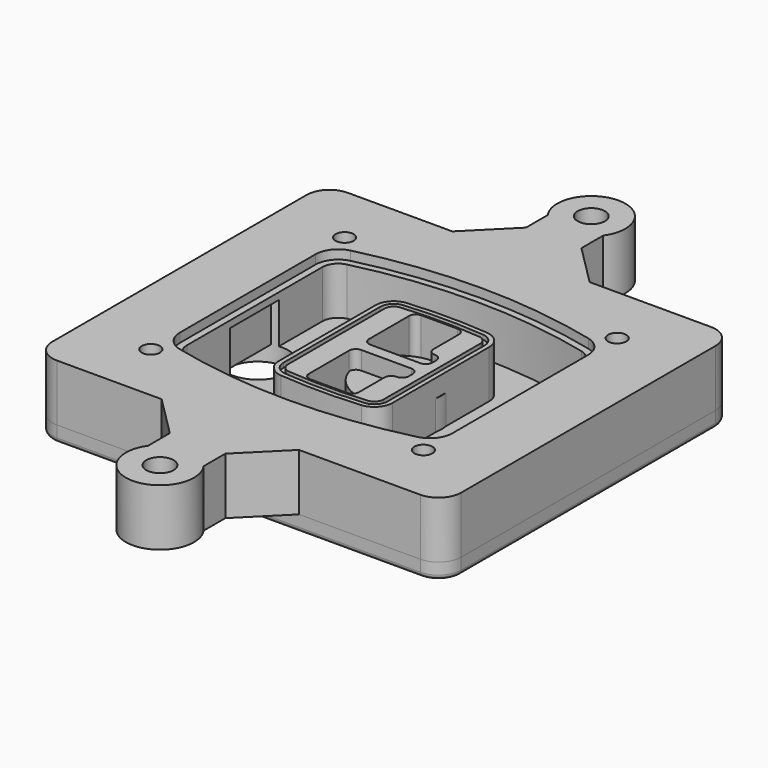
from build123d import *

# Parameters (mm, degrees)
F0_R      = 4
F1_DEPTH  = 25
F2_DEPTH  = 3
F3_DEPTH  = 18
F5_DEPTH  = 21
F6_DEPTH  = 2
F8_DEPTH  = 20
F9_DEPTH  = 16
F10_DEPTH = 25
F7_R      = 6
F7_R_2    = 4
F11_DEPTH = 6
F15_R     = 2
F16_R     = 4
F16_R_2   = 6
F17_DEPTH = 25
F18_DEPTH = 25
F19_DEPTH = 25


# Not quite as in the source:
# - a feature of the source that left no trace in its solid (it failed there, or was rolled back) is left out


with BuildPart() as f1:
    # F0 (on Top) → F1 (new body)
    with BuildSketch(Plane.XY):
        with BuildLine():
            ThreePointArc((-90, -70), (-87.0710678119, -77.0710678119), (-80, -80))
            Line((-80, -80), (80, -80))
            ThreePointArc((80, -80), (87.0710678119, -77.0710678119), (90, -70))
            Line((90, -70), (90, 70))
            ThreePointArc((90, 70), (87.0710678119, 77.0710678119), (80, 80))
            Line((80, 80), (-80, 80))
            ThreePointArc((-80, 80), (-87.0710678119, 77.0710678119), (-90, 70))
            Line((-90, 70), (-90, -70))
        make_face()
        with Locations((-60, -53.3333333333)):
            Circle(F0_R, mode=Mode.SUBTRACT)
        with Locations((60, -53.3333333333)):
            Circle(F0_R, mode=Mode.SUBTRACT)
        with Locations((-60, 53.3333333333)):
            Circle(F0_R, mode=Mode.SUBTRACT)
        with BuildLine():
            ThreePointArc((-64, 37.2990447398), (-61.0143011354, 45.9411029726), (-53.3306899286, 50.8970778549))
            ThreePointArc((-53.3306899286, 50.8970778549), (0, 57.3333333333), (53.3306899286, 50.8970778549))
            ThreePointArc((53.3306899286, 50.8970778549), (61.0143011354, 45.9411029726), (64, 37.2990447398))
            Line((64, 37.2990447398), (64, -37.2990447398))
            ThreePointArc((64, -37.2990447398), (61.0143011354, -45.9411029726), (53.3306899286, -50.8970778549))
            ThreePointArc((53.3306899286, -50.8970778549), (0, -57.3333333333), (-53.3306899286, -50.8970778549))
            ThreePointArc((-53.3306899286, -50.8970778549), (-61.0143011354, -45.9411029726), (-64, -37.2990447398))
            Line((-64, -37.2990447398), (-64, 37.2990447398))
        make_face(mode=Mode.SUBTRACT)
        with Locations((60, 53.3333333333)):
            Circle(F0_R, mode=Mode.SUBTRACT)
        with BuildLine():
            ThreePointArc((53.3306899286, 50.8970778549), (0, 57.3333333333), (-53.3306899286, 50.8970778549))
            ThreePointArc((-53.3306899286, 50.8970778549), (-61.0143011354, 45.9411029726), (-64, 37.2990447398))
            Line((-64, 37.2990447398), (-64, -37.2990447398))
            ThreePointArc((-64, -37.2990447398), (-61.0143011354, -45.9411029726), (-53.3306899286, -50.8970778549))
            ThreePointArc((-53.3306899286, -50.8970778549), (0, -57.3333333333), (53.3306899286, -50.8970778549))
            ThreePointArc((53.3306899286, -50.8970778549), (61.0143011354, -45.9411029726), (64, -37.2990447398))
            Line((64, -37.2990447398), (64, 37.2990447398))
            ThreePointArc((64, 37.2990447398), (61.0143011354, 45.9411029726), (53.3306899286, 50.8970778549))
        make_face()
        with BuildLine():
            Line((-60, -37.2990447398), (-60, 37.2990447398))
            ThreePointArc((-60, 37.2990447398), (-57.8673579538, 43.4719434775), (-52.3790642347, 47.0119255363))
            ThreePointArc((-52.3790642347, 47.0119255363), (0, 53.3333333333), (52.3790642347, 47.0119255363))
            ThreePointArc((52.3790642347, 47.0119255363), (57.8673579538, 43.4719434775), (60, 37.2990447398))
            Line((60, 37.2990447398), (60, -37.2990447398))
            ThreePointArc((60, -37.2990447398), (57.8673579538, -43.4719434775), (52.3790642347, -47.0119255363))
            ThreePointArc((52.3790642347, -47.0119255363), (0, -53.3333333333), (-52.3790642347, -47.0119255363))
            ThreePointArc((-52.3790642347, -47.0119255363), (-57.8673579538, -43.4719434775), (-60, -37.2990447398))
        make_face(mode=Mode.SUBTRACT)
        with BuildLine():
            ThreePointArc((-52.3790642347, 47.0119255363), (-57.8673579538, 43.4719434775), (-60, 37.2990447398))
            Line((-60, 37.2990447398), (-60, -37.2990447398))
            ThreePointArc((-60, -37.2990447398), (-57.8673579538, -43.4719434775), (-52.3790642347, -47.0119255363))
            ThreePointArc((-52.3790642347, -47.0119255363), (0, -53.3333333333), (52.3790642347, -47.0119255363))
            ThreePointArc((52.3790642347, -47.0119255363), (57.8673579538, -43.4719434775), (60, -37.2990447398))
            Line((60, -37.2990447398), (60, 37.2990447398))
            ThreePointArc((60, 37.2990447398), (57.8673579538, 43.4719434775), (52.3790642347, 47.0119255363))
            ThreePointArc((52.3790642347, 47.0119255363), (0, 53.3333333333), (-52.3790642347, 47.0119255363))
        make_face()
        with BuildLine():
            ThreePointArc((51.6653449643, 44.0980612973), (55.5071505677, 41.6200738562), (57, 37.2990447398))
            Line((57, 37.2990447398), (57, -37.2990447398))
            ThreePointArc((57, -37.2990447398), (55.5071505677, -41.6200738562), (51.6653449643, -44.0980612973))
            ThreePointArc((51.6653449643, -44.0980612973), (0, -50.3333333333), (-51.6653449643, -44.0980612973))
            ThreePointArc((-51.6653449643, -44.0980612973), (-55.5071505677, -41.6200738562), (-57, -37.2990447398))
            Line((-57, -37.2990447398), (-57, 37.2990447398))
            ThreePointArc((-57, 37.2990447398), (-55.5071505677, 41.6200738562), (-51.6653449643, 44.0980612973))
            ThreePointArc((-51.6653449643, 44.0980612973), (0, 50.3333333333), (51.6653449643, 44.0980612973))
        make_face(mode=Mode.SUBTRACT)
        with BuildLine():
            Line((57, -37.2990447398), (57, 37.2990447398))
            ThreePointArc((57, 37.2990447398), (55.5071505677, 41.6200738562), (51.6653449643, 44.0980612973))
            ThreePointArc((51.6653449643, 44.0980612973), (0, 50.3333333333), (-51.6653449643, 44.0980612973))
            ThreePointArc((-51.6653449643, 44.0980612973), (-55.5071505677, 41.6200738562), (-57, 37.2990447398))
            Line((-57, 37.2990447398), (-57, -37.2990447398))
            ThreePointArc((-57, -37.2990447398), (-55.5071505677, -41.6200738562), (-51.6653449643, -44.0980612973))
            ThreePointArc((-51.6653449643, -44.0980612973), (0, -50.3333333333), (51.6653449643, -44.0980612973))
            ThreePointArc((51.6653449643, -44.0980612973), (55.5071505677, -41.6200738562), (57, -37.2990447398))
        make_face()
    extrude(amount=-F1_DEPTH)

    # F0 (on Top) → F2 (join)
    with BuildSketch(Plane.XY):
        with BuildLine():
            ThreePointArc((-52.3790642347, 47.0119255363), (-57.8673579538, 43.4719434775), (-60, 37.2990447398))
            Line((-60, 37.2990447398), (-60, -37.2990447398))
            ThreePointArc((-60, -37.2990447398), (-57.8673579538, -43.4719434775), (-52.3790642347, -47.0119255363))
            ThreePointArc((-52.3790642347, -47.0119255363), (0, -53.3333333333), (52.3790642347, -47.0119255363))
            ThreePointArc((52.3790642347, -47.0119255363), (57.8673579538, -43.4719434775), (60, -37.2990447398))
            Line((60, -37.2990447398), (60, 37.2990447398))
            ThreePointArc((60, 37.2990447398), (57.8673579538, 43.4719434775), (52.3790642347, 47.0119255363))
            ThreePointArc((52.3790642347, 47.0119255363), (0, 53.3333333333), (-52.3790642347, 47.0119255363))
        make_face()
        with BuildLine():
            ThreePointArc((51.6653449643, 44.0980612973), (55.5071505677, 41.6200738562), (57, 37.2990447398))
            Line((57, 37.2990447398), (57, -37.2990447398))
            ThreePointArc((57, -37.2990447398), (55.5071505677, -41.6200738562), (51.6653449643, -44.0980612973))
            ThreePointArc((51.6653449643, -44.0980612973), (0, -50.3333333333), (-51.6653449643, -44.0980612973))
            ThreePointArc((-51.6653449643, -44.0980612973), (-55.5071505677, -41.6200738562), (-57, -37.2990447398))
            Line((-57, -37.2990447398), (-57, 37.2990447398))
            ThreePointArc((-57, 37.2990447398), (-55.5071505677, 41.6200738562), (-51.6653449643, 44.0980612973))
            ThreePointArc((-51.6653449643, 44.0980612973), (0, 50.3333333333), (51.6653449643, 44.0980612973))
        make_face(mode=Mode.SUBTRACT)
    extrude(amount=F2_DEPTH)

    # F0 (on Top) → F3 (cut)
    with BuildSketch(Plane.XY):
        with BuildLine():
            Line((57, -37.2990447398), (57, 37.2990447398))
            ThreePointArc((57, 37.2990447398), (55.5071505677, 41.6200738562), (51.6653449643, 44.0980612973))
            ThreePointArc((51.6653449643, 44.0980612973), (0, 50.3333333333), (-51.6653449643, 44.0980612973))
            ThreePointArc((-51.6653449643, 44.0980612973), (-55.5071505677, 41.6200738562), (-57, 37.2990447398))
            Line((-57, 37.2990447398), (-57, -37.2990447398))
            ThreePointArc((-57, -37.2990447398), (-55.5071505677, -41.6200738562), (-51.6653449643, -44.0980612973))
            ThreePointArc((-51.6653449643, -44.0980612973), (0, -50.3333333333), (51.6653449643, -44.0980612973))
            ThreePointArc((51.6653449643, -44.0980612973), (55.5071505677, -41.6200738562), (57, -37.2990447398))
        make_face()
    extrude(amount=-F3_DEPTH, mode=Mode.SUBTRACT)

    # F4 (on face) → F5 (join, through all)
    with BuildSketch(Plane.XY.offset(3)):
        with BuildLine():
            ThreePointArc((-25, -26.587695628), (-22.8992979869, -31.9912392117), (-17.7004291845, -34.5569740744))
            ThreePointArc((-17.7004291845, -34.5569740744), (0, -35.3333333333), (17.7004291845, -34.5569740744))
            ThreePointArc((17.7004291845, -34.5569740744), (22.8992979869, -31.9912392117), (25, -26.587695628))
            Line((25, -26.587695628), (25, 26.587695628))
            ThreePointArc((25, 26.587695628), (22.8992979869, 31.9912392117), (17.7004291845, 34.5569740744))
            ThreePointArc((17.7004291845, 34.5569740744), (0, 35.3333333333), (-17.7004291845, 34.5569740744))
            ThreePointArc((-17.7004291845, 34.5569740744), (-22.8992979869, 31.9912392117), (-25, 26.587695628))
            Line((-25, 26.587695628), (-25, -26.587695628))
        make_face()
        with BuildLine():
            ThreePointArc((17.5253218884, 32.5646544628), (21.4244734902, 30.6403533158), (23, 26.587695628))
            Line((23, 26.587695628), (23, -26.587695628))
            ThreePointArc((23, -26.587695628), (21.4244734902, -30.6403533158), (17.5253218884, -32.5646544628))
            ThreePointArc((17.5253218884, -32.5646544628), (0, -33.3333333333), (-17.5253218884, -32.5646544628))
            ThreePointArc((-17.5253218884, -32.5646544628), (-21.4244734902, -30.6403533158), (-23, -26.587695628))
            Line((-23, -26.587695628), (-23, 26.587695628))
            ThreePointArc((-23, 26.587695628), (-21.4244734902, 30.6403533158), (-17.5253218884, 32.5646544628))
            ThreePointArc((-17.5253218884, 32.5646544628), (0, 33.3333333333), (17.5253218884, 32.5646544628))
        make_face(mode=Mode.SUBTRACT)
        with BuildLine():
            Line((23, -26.587695628), (23, 26.587695628))
            ThreePointArc((23, 26.587695628), (21.4244734902, 30.6403533158), (17.5253218884, 32.5646544628))
            ThreePointArc((17.5253218884, 32.5646544628), (0, 33.3333333333), (-17.5253218884, 32.5646544628))
            ThreePointArc((-17.5253218884, 32.5646544628), (-21.4244734902, 30.6403533158), (-23, 26.587695628))
            Line((-23, 26.587695628), (-23, -26.587695628))
            ThreePointArc((-23, -26.587695628), (-21.4244734902, -30.6403533158), (-17.5253218884, -32.5646544628))
            ThreePointArc((-17.5253218884, -32.5646544628), (0, -33.3333333333), (17.5253218884, -32.5646544628))
            ThreePointArc((17.5253218884, -32.5646544628), (21.4244734902, -30.6403533158), (23, -26.587695628))
        make_face()
        with BuildLine():
            ThreePointArc((17.3502145923, 30.5723348512), (19.9496489934, 29.2894674198), (21, 26.587695628))
            Line((21, 26.587695628), (21, -26.587695628))
            ThreePointArc((21, -26.587695628), (19.9496489934, -29.2894674198), (17.3502145923, -30.5723348512))
            ThreePointArc((17.3502145923, -30.5723348512), (0, -31.3333333333), (-17.3502145923, -30.5723348512))
            ThreePointArc((-17.3502145923, -30.5723348512), (-19.9496489934, -29.2894674198), (-21, -26.587695628))
            Line((-21, -26.587695628), (-21, 26.587695628))
            ThreePointArc((-21, 26.587695628), (-19.9496489934, 29.2894674198), (-17.3502145923, 30.5723348512))
            ThreePointArc((-17.3502145923, 30.5723348512), (0, 31.3333333333), (17.3502145923, 30.5723348512))
        make_face(mode=Mode.SUBTRACT)
        with BuildLine():
            Line((21, -26.587695628), (21, 26.587695628))
            ThreePointArc((21, 26.587695628), (19.9496489934, 29.2894674198), (17.3502145923, 30.5723348512))
            ThreePointArc((17.3502145923, 30.5723348512), (0, 31.3333333333), (-17.3502145923, 30.5723348512))
            ThreePointArc((-17.3502145923, 30.5723348512), (-19.9496489934, 29.2894674198), (-21, 26.587695628))
            Line((-21, 26.587695628), (-21, -26.587695628))
            ThreePointArc((-21, -26.587695628), (-19.9496489934, -29.2894674198), (-17.3502145923, -30.5723348512))
            ThreePointArc((-17.3502145923, -30.5723348512), (0, -31.3333333333), (17.3502145923, -30.5723348512))
            ThreePointArc((17.3502145923, -30.5723348512), (19.9496489934, -29.2894674198), (21, -26.587695628))
        make_face()
        with BuildLine():
            Line((-8, -2.5), (14, -2.5))
            ThreePointArc((14, -2.5), (16.1213203436, -3.3786796564), (17, -5.5))
            Line((17, -5.5), (17, -7.5))
            ThreePointArc((17, -7.5), (16.1213203436, -9.6213203436), (14, -10.5))
            ThreePointArc((14, -10.5), (11.8786796564, -11.3786796564), (11, -13.5))
            Line((11, -13.5), (11, -27.5))
            ThreePointArc((11, -27.5), (10.1213203436, -29.6213203436), (8, -30.5))
            Line((8, -30.5), (-8, -30.5))
            ThreePointArc((-8, -30.5), (-10.1213203436, -29.6213203436), (-11, -27.5))
            Line((-11, -27.5), (-11, -5.5))
            ThreePointArc((-11, -5.5), (-10.1213203436, -3.3786796564), (-8, -2.5))
        make_face(mode=Mode.SUBTRACT)
        with BuildLine():
            ThreePointArc((-8, 2.5), (-10.1213203436, 3.3786796564), (-11, 5.5))
            Line((-11, 5.5), (-11, 27.5))
            ThreePointArc((-11, 27.5), (-10.1213203436, 29.6213203436), (-8, 30.5))
            Line((-8, 30.5), (8, 30.5))
            ThreePointArc((8, 30.5), (10.1213203436, 29.6213203436), (11, 27.5))
            Line((11, 27.5), (11, 13.5))
            ThreePointArc((11, 13.5), (11.8786796564, 11.3786796564), (14, 10.5))
            ThreePointArc((14, 10.5), (16.1213203436, 9.6213203436), (17, 7.5))
            Line((17, 7.5), (17, 5.5))
            ThreePointArc((17, 5.5), (16.1213203436, 3.3786796564), (14, 2.5))
            Line((14, 2.5), (-8, 2.5))
        make_face(mode=Mode.SUBTRACT)
    extrude(amount=-F5_DEPTH)

    # F4 (on face) → F6 (cut)
    with BuildSketch(Plane.XY.offset(3)):
        with BuildLine():
            Line((23, -26.587695628), (23, 26.587695628))
            ThreePointArc((23, 26.587695628), (21.4244734902, 30.6403533158), (17.5253218884, 32.5646544628))
            ThreePointArc((17.5253218884, 32.5646544628), (0, 33.3333333333), (-17.5253218884, 32.5646544628))
            ThreePointArc((-17.5253218884, 32.5646544628), (-21.4244734902, 30.6403533158), (-23, 26.587695628))
            Line((-23, 26.587695628), (-23, -26.587695628))
            ThreePointArc((-23, -26.587695628), (-21.4244734902, -30.6403533158), (-17.5253218884, -32.5646544628))
            ThreePointArc((-17.5253218884, -32.5646544628), (0, -33.3333333333), (17.5253218884, -32.5646544628))
            ThreePointArc((17.5253218884, -32.5646544628), (21.4244734902, -30.6403533158), (23, -26.587695628))
        make_face()
        with BuildLine():
            ThreePointArc((17.3502145923, 30.5723348512), (19.9496489934, 29.2894674198), (21, 26.587695628))
            Line((21, 26.587695628), (21, -26.587695628))
            ThreePointArc((21, -26.587695628), (19.9496489934, -29.2894674198), (17.3502145923, -30.5723348512))
            ThreePointArc((17.3502145923, -30.5723348512), (0, -31.3333333333), (-17.3502145923, -30.5723348512))
            ThreePointArc((-17.3502145923, -30.5723348512), (-19.9496489934, -29.2894674198), (-21, -26.587695628))
            Line((-21, -26.587695628), (-21, 26.587695628))
            ThreePointArc((-21, 26.587695628), (-19.9496489934, 29.2894674198), (-17.3502145923, 30.5723348512))
            ThreePointArc((-17.3502145923, 30.5723348512), (0, 31.3333333333), (17.3502145923, 30.5723348512))
        make_face(mode=Mode.SUBTRACT)
    extrude(amount=-F6_DEPTH, mode=Mode.SUBTRACT)

    # F7 (on face) → F8 (join)
    with BuildSketch(Plane(origin=(0, 0, -25), x_dir=(1, 0, 0), z_dir=(0, 0, -1))):
        with BuildLine():
            ThreePointArc((-6.71157564, 0), (6.7567035675, 13.4682792075), (20.224982775, 0))
            Line((20.224982775, 0), (25.224982775, 0))
            ThreePointArc((25.224982775, 0), (6.7567035675, 18.4682792075), (-11.71157564, 0))
            Line((-11.71157564, 0), (-6.71157564, 0))
        make_face()
        with BuildLine():
            Line((-6.71157564, 0), (20.224982775, 0))
            ThreePointArc((20.224982775, 0), (6.7567035675, 13.4682792075), (-6.71157564, 0))
        make_face()
        with BuildLine():
            ThreePointArc((-6.71157564, 0), (6.7567035675, -13.4682792075), (20.224982775, 0))
            Line((20.224982775, 0), (-6.71157564, 0))
        make_face()
        with BuildLine():
            Line((25.224982775, 0), (20.224982775, 0))
            ThreePointArc((20.224982775, 0), (6.7567035675, -13.4682792075), (-6.71157564, 0))
            Line((-6.71157564, 0), (-11.71157564, 0))
            ThreePointArc((-11.71157564, 0), (6.7567035675, -18.4682792075), (25.224982775, 0))
        make_face()
    extrude(amount=-F8_DEPTH)

    # F7 (on face) → F9 (cut)
    with BuildSketch(Plane(origin=(0, 0, -25), x_dir=(1, 0, 0), z_dir=(0, 0, -1))):
        with BuildLine():
            Line((-6.71157564, 0), (20.224982775, 0))
            ThreePointArc((20.224982775, 0), (6.7567035675, 13.4682792075), (-6.71157564, 0))
        make_face()
        with BuildLine():
            ThreePointArc((-6.71157564, 0), (6.7567035675, -13.4682792075), (20.224982775, 0))
            Line((20.224982775, 0), (-6.71157564, 0))
        make_face()
    extrude(amount=-F9_DEPTH, mode=Mode.SUBTRACT)

    # F7 (on face) → F10 (cut)
    with BuildSketch(Plane(origin=(0, 0, -25), x_dir=(1, 0, 0), z_dir=(0, 0, -1))):
        with BuildLine():
            Line((-69.0318229325, 0), (-42.0952645175, 0))
            ThreePointArc((-42.0952645175, 0), (-55.563543725, 13.4682792075), (-69.0318229325, 0))
        make_face()
        with BuildLine():
            ThreePointArc((-69.0318229325, 0), (-55.563543725, -13.4682792075), (-42.0952645175, 0))
            Line((-42.0952645175, 0), (-69.0318229325, 0))
        make_face()
    extrude(amount=-F10_DEPTH, mode=Mode.SUBTRACT)

    # F7 (on face) → F11 (cut)
    with BuildSketch(Plane(origin=(0, 0, -25), x_dir=(1, 0, 0), z_dir=(0, 0, -1))):
        with Locations((60, -53.3333333333)):
            Circle(F7_R)
        with Locations((60, -53.3333333333)):
            Circle(F7_R_2, mode=Mode.SUBTRACT)
        with Locations((-60, -53.3333333333)):
            Circle(F7_R)
        with Locations((-60, -53.3333333333)):
            Circle(F7_R_2, mode=Mode.SUBTRACT)
        with Locations((-60, 53.3333333333)):
            Circle(F7_R)
        with Locations((-60, 53.3333333333)):
            Circle(F7_R_2, mode=Mode.SUBTRACT)
        with Locations((60, 53.3333333333)):
            Circle(F7_R)
        with Locations((60, 53.3333333333)):
            Circle(F7_R_2, mode=Mode.SUBTRACT)
    extrude(amount=-F11_DEPTH, mode=Mode.SUBTRACT)

    # F15
    f15_edges = [f1.edges().sort_by_distance(p)[0] for p in [
        (0, -80, -25),
        (-87.071068, -77.071068, -25),
        (-90, 0, -25),
        (-87.071068, 77.071068, -25),
        (87.071068, -77.071068, -25),
        (0, 80, -25),
        (90, 0, -25),
        (87.071068, 77.071068, -25),
    ]]
    fillet(f15_edges, radius=F15_R)


with BuildPart() as f17:
    # F16 (on face) → F17 (new body)
    with BuildSketch(Plane.XY.offset(-18)):
        with BuildLine():
            Line((-33.9034107223, 80), (-80, 80))
            ThreePointArc((-80, 80), (-87.0710678119, 77.0710678119), (-90, 70))
            Line((-90, 70), (-90, -70))
            ThreePointArc((-90, -70), (-87.0710678119, -77.0710678119), (-80, -80))
            Line((-80, -80), (-33.9034107223, -80))
            Line((-33.9034107223, -80), (26.53131634, -80))
            Line((26.53131634, -80), (80, -80))
            ThreePointArc((80, -80), (87.0710678119, -77.0710678119), (90, -70))
            Line((90, -70), (90, 70))
            ThreePointArc((90, 70), (87.0710678119, 77.0710678119), (80, 80))
            Line((80, 80), (26.53131634, 80))
            Line((26.53131634, 80), (-33.9034107223, 80))
        make_face()
        with Locations((-60, -53.3333333333)):
            Circle(F16_R, mode=Mode.SUBTRACT)
        with Locations((60, -53.3333333333)):
            Circle(F16_R, mode=Mode.SUBTRACT)
        with Locations((-60, 53.3333333333)):
            Circle(F16_R, mode=Mode.SUBTRACT)
        with BuildLine():
            ThreePointArc((-52.3790642347, 47.0119255363), (0, 53.3333333333), (52.3790642347, 47.0119255363))
            ThreePointArc((52.3790642347, 47.0119255363), (57.8673579538, 43.4719434775), (60, 37.2990447398))
            Line((60, 37.2990447398), (60, -37.2990447398))
            ThreePointArc((60, -37.2990447398), (57.8673579538, -43.4719434775), (52.3790642347, -47.0119255363))
            ThreePointArc((52.3790642347, -47.0119255363), (0, -53.3333333333), (-52.3790642347, -47.0119255363))
            ThreePointArc((-52.3790642347, -47.0119255363), (-57.8673579538, -43.4719434775), (-60, -37.2990447398))
            Line((-60, -37.2990447398), (-60, 37.2990447398))
            ThreePointArc((-60, 37.2990447398), (-57.8673579538, 43.4719434775), (-52.3790642347, 47.0119255363))
        make_face(mode=Mode.SUBTRACT)
        with Locations((60, 53.3333333333)):
            Circle(F16_R, mode=Mode.SUBTRACT)
        with BuildLine():
            Line((-15.9034107223, 98), (-33.9034107223, 80))
            Line((-33.9034107223, 80), (26.53131634, 80))
            Line((26.53131634, 80), (8.53131634, 98))
            Line((8.53131634, 98), (8.53131634, 110))
            ThreePointArc((8.53131634, 110), (-3.6860471911, 133.7026449054), (-15.9034107223, 110))
            Line((-15.9034107223, 110), (-15.9034107223, 98))
        make_face()
        with Locations((-3.6860471911, 118.7026449054)):
            Circle(F16_R_2, mode=Mode.SUBTRACT)
        with BuildLine():
            Line((26.53131634, -80), (-33.9034107223, -80))
            Line((-33.9034107223, -80), (-15.9034107223, -98))
            Line((-15.9034107223, -98), (-15.9034107223, -110))
            ThreePointArc((-15.9034107223, -110), (-3.6860471911, -133.7026449054), (8.53131634, -110))
            Line((8.53131634, -110), (8.53131634, -98))
            Line((8.53131634, -98), (26.53131634, -80))
        make_face()
        with Locations((-3.6860471911, -118.7026449054)):
            Circle(F16_R_2, mode=Mode.SUBTRACT)
    extrude(amount=F17_DEPTH)


with BuildPart() as f18:
    # F16 (on face) → F18 (new body)
    with BuildSketch(Plane.XY.offset(-18)):
        with BuildLine():
            Line((-33.9034107223, 80), (-80, 80))
            ThreePointArc((-80, 80), (-87.0710678119, 77.0710678119), (-90, 70))
            Line((-90, 70), (-90, -70))
            ThreePointArc((-90, -70), (-87.0710678119, -77.0710678119), (-80, -80))
            Line((-80, -80), (-33.9034107223, -80))
            Line((-33.9034107223, -80), (26.53131634, -80))
            Line((26.53131634, -80), (80, -80))
            ThreePointArc((80, -80), (87.0710678119, -77.0710678119), (90, -70))
            Line((90, -70), (90, 70))
            ThreePointArc((90, 70), (87.0710678119, 77.0710678119), (80, 80))
            Line((80, 80), (26.53131634, 80))
            Line((26.53131634, 80), (-33.9034107223, 80))
        make_face()
        with Locations((-60, -53.3333333333)):
            Circle(F16_R, mode=Mode.SUBTRACT)
        with Locations((60, -53.3333333333)):
            Circle(F16_R, mode=Mode.SUBTRACT)
        with Locations((-60, 53.3333333333)):
            Circle(F16_R, mode=Mode.SUBTRACT)
        with BuildLine():
            ThreePointArc((-52.3790642347, 47.0119255363), (0, 53.3333333333), (52.3790642347, 47.0119255363))
            ThreePointArc((52.3790642347, 47.0119255363), (57.8673579538, 43.4719434775), (60, 37.2990447398))
            Line((60, 37.2990447398), (60, -37.2990447398))
            ThreePointArc((60, -37.2990447398), (57.8673579538, -43.4719434775), (52.3790642347, -47.0119255363))
            ThreePointArc((52.3790642347, -47.0119255363), (0, -53.3333333333), (-52.3790642347, -47.0119255363))
            ThreePointArc((-52.3790642347, -47.0119255363), (-57.8673579538, -43.4719434775), (-60, -37.2990447398))
            Line((-60, -37.2990447398), (-60, 37.2990447398))
            ThreePointArc((-60, 37.2990447398), (-57.8673579538, 43.4719434775), (-52.3790642347, 47.0119255363))
        make_face(mode=Mode.SUBTRACT)
        with Locations((60, 53.3333333333)):
            Circle(F16_R, mode=Mode.SUBTRACT)
        with BuildLine():
            Line((-15.9034107223, 98), (-33.9034107223, 80))
            Line((-33.9034107223, 80), (26.53131634, 80))
            Line((26.53131634, 80), (8.53131634, 98))
            Line((8.53131634, 98), (8.53131634, 110))
            ThreePointArc((8.53131634, 110), (-3.6860471911, 133.7026449054), (-15.9034107223, 110))
            Line((-15.9034107223, 110), (-15.9034107223, 98))
        make_face()
        with Locations((-3.6860471911, 118.7026449054)):
            Circle(F16_R_2, mode=Mode.SUBTRACT)
        with BuildLine():
            Line((26.53131634, -80), (-33.9034107223, -80))
            Line((-33.9034107223, -80), (-15.9034107223, -98))
            Line((-15.9034107223, -98), (-15.9034107223, -110))
            ThreePointArc((-15.9034107223, -110), (-3.6860471911, -133.7026449054), (8.53131634, -110))
            Line((8.53131634, -110), (8.53131634, -98))
            Line((8.53131634, -98), (26.53131634, -80))
        make_face()
        with Locations((-3.6860471911, -118.7026449054)):
            Circle(F16_R_2, mode=Mode.SUBTRACT)
    extrude(amount=F18_DEPTH)


with BuildPart() as f19:
    # F16 (on face) → F19 (new body)
    with BuildSketch(Plane.XY.offset(-18)):
        with BuildLine():
            Line((-33.9034107223, 80), (-80, 80))
            ThreePointArc((-80, 80), (-87.0710678119, 77.0710678119), (-90, 70))
            Line((-90, 70), (-90, -70))
            ThreePointArc((-90, -70), (-87.0710678119, -77.0710678119), (-80, -80))
            Line((-80, -80), (-33.9034107223, -80))
            Line((-33.9034107223, -80), (26.53131634, -80))
            Line((26.53131634, -80), (80, -80))
            ThreePointArc((80, -80), (87.0710678119, -77.0710678119), (90, -70))
            Line((90, -70), (90, 70))
            ThreePointArc((90, 70), (87.0710678119, 77.0710678119), (80, 80))
            Line((80, 80), (26.53131634, 80))
            Line((26.53131634, 80), (-33.9034107223, 80))
        make_face()
        with Locations((-60, -53.3333333333)):
            Circle(F16_R, mode=Mode.SUBTRACT)
        with Locations((60, -53.3333333333)):
            Circle(F16_R, mode=Mode.SUBTRACT)
        with Locations((-60, 53.3333333333)):
            Circle(F16_R, mode=Mode.SUBTRACT)
        with BuildLine():
            ThreePointArc((-52.3790642347, 47.0119255363), (0, 53.3333333333), (52.3790642347, 47.0119255363))
            ThreePointArc((52.3790642347, 47.0119255363), (57.8673579538, 43.4719434775), (60, 37.2990447398))
            Line((60, 37.2990447398), (60, -37.2990447398))
            ThreePointArc((60, -37.2990447398), (57.8673579538, -43.4719434775), (52.3790642347, -47.0119255363))
            ThreePointArc((52.3790642347, -47.0119255363), (0, -53.3333333333), (-52.3790642347, -47.0119255363))
            ThreePointArc((-52.3790642347, -47.0119255363), (-57.8673579538, -43.4719434775), (-60, -37.2990447398))
            Line((-60, -37.2990447398), (-60, 37.2990447398))
            ThreePointArc((-60, 37.2990447398), (-57.8673579538, 43.4719434775), (-52.3790642347, 47.0119255363))
        make_face(mode=Mode.SUBTRACT)
        with Locations((60, 53.3333333333)):
            Circle(F16_R, mode=Mode.SUBTRACT)
        with BuildLine():
            Line((-15.9034107223, 98), (-33.9034107223, 80))
            Line((-33.9034107223, 80), (26.53131634, 80))
            Line((26.53131634, 80), (8.53131634, 98))
            Line((8.53131634, 98), (8.53131634, 110))
            ThreePointArc((8.53131634, 110), (-3.6860471911, 133.7026449054), (-15.9034107223, 110))
            Line((-15.9034107223, 110), (-15.9034107223, 98))
        make_face()
        with Locations((-3.6860471911, 118.7026449054)):
            Circle(F16_R_2, mode=Mode.SUBTRACT)
        with BuildLine():
            Line((26.53131634, -80), (-33.9034107223, -80))
            Line((-33.9034107223, -80), (-15.9034107223, -98))
            Line((-15.9034107223, -98), (-15.9034107223, -110))
            ThreePointArc((-15.9034107223, -110), (-3.6860471911, -133.7026449054), (8.53131634, -110))
            Line((8.53131634, -110), (8.53131634, -98))
            Line((8.53131634, -98), (26.53131634, -80))
        make_face()
        with Locations((-3.6860471911, -118.7026449054)):
            Circle(F16_R_2, mode=Mode.SUBTRACT)
    extrude(amount=F19_DEPTH)


solid = Compound([f1.part, f17.part, f18.part, f19.part])
